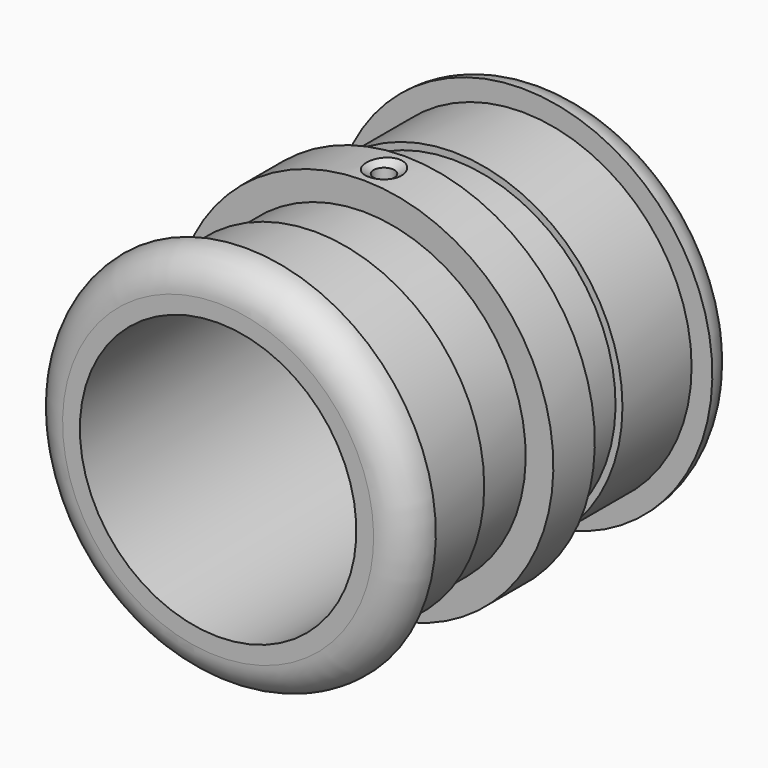
from build123d import *

# Parameters (mm, degrees)
F4_R = 9.99999


# Not quite as in the source:
# - a fillet or chamfer is up to 0.001 mm smaller than in the source, because OpenCascade refuses the exact size


with BuildPart() as f1:
    # F0 (on Right) → F1 (revolve)
    with BuildSketch(Plane.YZ):
        Polygon((-60, 55), (-60, 40), (60, 40), (60, 55), (50, 55), (50, 49), (25, 49), (25, 47), (7.5, 47), (7.5, 55), (-7.5, 55), (-7.5, 47), (-25, 47), (-25, 49), (-50, 49), (-50, 55), align=None)
    revolve(axis=Axis((0, -7.7097125049, 0), (0, 1, 0)))

    # F2 (on Right) → F3 (revolve, cut)
    with BuildSketch(Plane.YZ):
        Polygon((7.2320508076, 56), (0, 56), (0, 36), (3, 36), (3, 53.556624327), align=None)
    revolve(axis=Axis((0, 0, 50.0545714922), (0, 0, -1)), mode=Mode.SUBTRACT)

    # F4 (radius 10 in the source; OpenCascade refuses exactly that, so slightly less here)
    f4_edges = [f1.edges().sort_by_distance(p)[0] for p in [
        (0, 60, -55),
        (0, -60, -55),
    ]]
    fillet(f4_edges, radius=F4_R)


solid = f1.part
